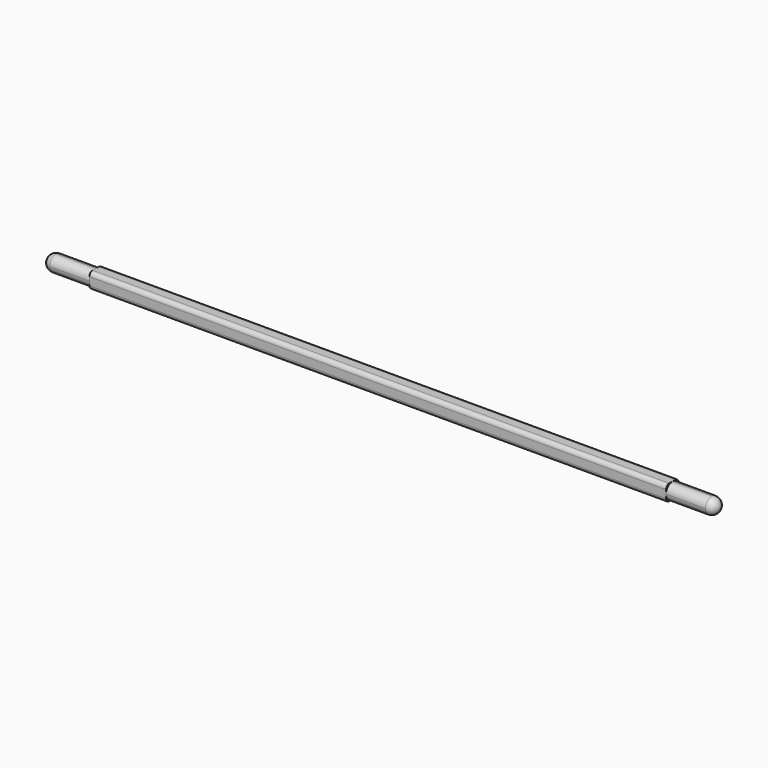
from build123d import *

# Parameters (mm, degrees)
F0_W     = 146
F0_H     = 4
F1_DEPTH = 4
F3_DEPTH = 12
F6_DEPTH = 12
F8_R     = 1


# Not quite as in the source:
# - a fillet or chamfer that OpenCascade refuses, or shapes differently, is made with other operations: its cross-section is extruded or revolved along the edge and cut away or added


with BuildPart() as f1:
    # F0 (on Top) → F1 (new body)
    with BuildSketch(Plane.XY):
        Rectangle(F0_W, F0_H)
    extrude(amount=F1_DEPTH)

    # F2 (on face) → F3 (join)
    with BuildSketch(Plane(origin=(-73, 0, 0), x_dir=(0, -1, 0), z_dir=(-1, 0, 0))):
        with BuildLine():
            ThreePointArc((0, 0), (1.4142135624, 0.5857864376), (2, 2))
            ThreePointArc((2, 2), (1.4142135624, 3.4142135624), (0, 4))
            ThreePointArc((0, 4), (-1.4142135624, 3.4142135624), (-2, 2))
            ThreePointArc((-2, 2), (-1.4142135624, 0.5857864376), (0, 0))
        make_face()
    extrude(amount=F3_DEPTH)

    # F4: fillet of radius 2 on 1 edges, made by hand

    # F4_s1 → F4_t2 (revolve, cut)
    with BuildSketch(Plane.XZ):
        with BuildLine():
            ThreePointArc((-83, 0), (-84.4142135624, 0.5857864376), (-85, 2))
            Line((-85, 2), (-85, 0))
            Line((-85, 0), (-83, 0))
        make_face()
    revolve(axis=Axis((-85, 0, 2), (1, 0, 0)), mode=Mode.SUBTRACT)

    # F5 (on face) → F6 (join)
    with BuildSketch(Plane.YZ.offset(73)):
        with BuildLine():
            ThreePointArc((0, 0), (1.4142135624, 0.5857864376), (2, 2))
            ThreePointArc((2, 2), (1.4142135624, 3.4142135624), (0, 4))
            ThreePointArc((0, 4), (-1.4142135624, 3.4142135624), (-2, 2))
            ThreePointArc((-2, 2), (-1.4142135624, 0.5857864376), (0, 0))
        make_face()
    extrude(amount=F6_DEPTH)

    # F7: fillet of radius 2 on 1 edges, made by hand

    # F7_s1 → F7_t2 (revolve, cut)
    with BuildSketch(Plane.XZ):
        with BuildLine():
            ThreePointArc((83, 0), (84.4142135624, 0.5857864376), (85, 2))
            Line((85, 2), (85, 0))
            Line((85, 0), (83, 0))
        make_face()
    revolve(axis=Axis((85, 0, 2), (-1, 0, 0)), mode=Mode.SUBTRACT)

    # F8
    f8_edges = [f1.edges().sort_by_distance(p)[0] for p in [
        (0, -2, 4),
        (0, -2, 0),
        (0, 2, 0),
        (0, 2, 4),
    ]]
    fillet(f8_edges, radius=F8_R)


solid = f1.part
